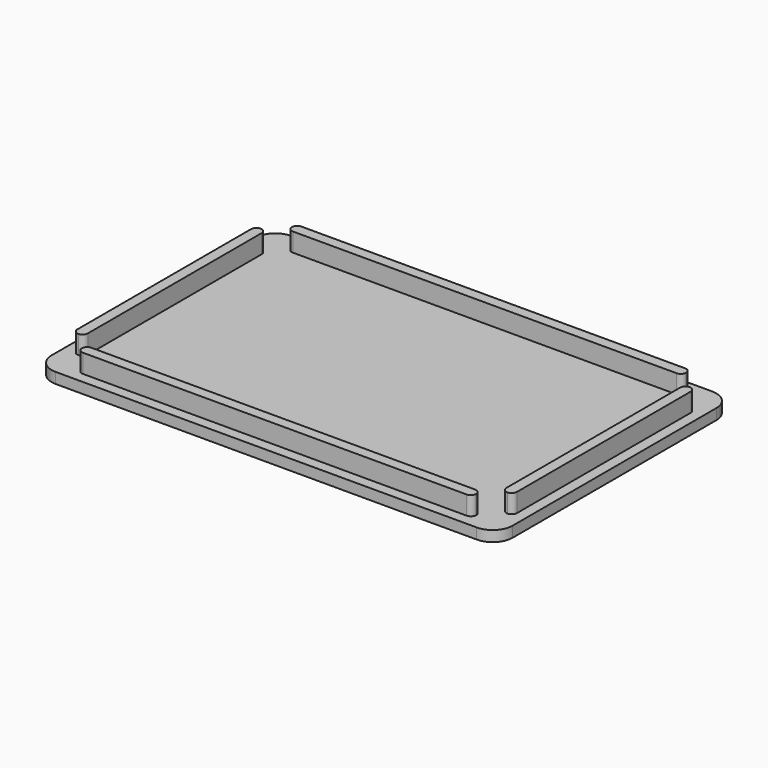
from build123d import *

# Parameters (mm, degrees)
F0_W     = 69.2
F0_H     = 44.2
F1_DEPTH = 1.6
F2_W     = 59.2
F2_H     = 1.6
F2_W_2   = 1.6
F2_H_2   = 34.2
F3_DEPTH = 2.8
F4_R     = 3
F5_R     = 0.79999


# Not quite as in the source:
# - a fillet or chamfer is up to 0.001 mm smaller than in the source, because OpenCascade refuses the exact size


with BuildPart() as f1:
    # F0 (on Top) → F1 (new body)
    with BuildSketch(Plane.XY):
        Rectangle(F0_W, F0_H)
    extrude(amount=F1_DEPTH)

    # F2 (on face) → F3 (join)
    with BuildSketch(Plane.XY.offset(1.6)):
        with Locations((0, -19.7)):
            Rectangle(F2_W, F2_H)
        with Locations((-32.2, 0)):
            Rectangle(F2_W_2, F2_H_2)
        with Locations((32.2, 0)):
            Rectangle(F2_W_2, F2_H_2)
        with Locations((0, 19.7)):
            Rectangle(F2_W, F2_H)
    extrude(amount=F3_DEPTH)

    # F4
    f4_edges = [f1.edges().sort_by_distance(p)[0] for p in [
        (34.6, -22.1, 0.8),
        (34.6, 22.1, 0.8),
        (-34.6, -22.1, 0.8),
        (-34.6, 22.1, 0.8),
    ]]
    fillet(f4_edges, radius=F4_R)

    # F5 (radius 0.8 in the source; OpenCascade refuses exactly that, so slightly less here)
    f5_edges = [f1.edges().sort_by_distance(p)[0] for p in [
        (29.6, -20.5, 3),
        (29.6, -18.9, 3),
        (33, -17.1, 3),
        (31.4, -17.1, 3),
        (29.6, 18.9, 3),
        (29.6, 20.5, 3),
        (-33, -17.1, 3),
        (-31.4, 17.1, 3),
        (-31.4, -17.1, 3),
        (-29.6, 18.9, 3),
        (31.4, 17.1, 3),
        (33, 17.1, 3),
        (-33, 17.1, 3),
        (-29.6, -18.9, 3),
        (-29.6, 20.5, 3),
        (-29.6, -20.5, 3),
    ]]
    fillet(f5_edges, radius=F5_R)


solid = f1.part
